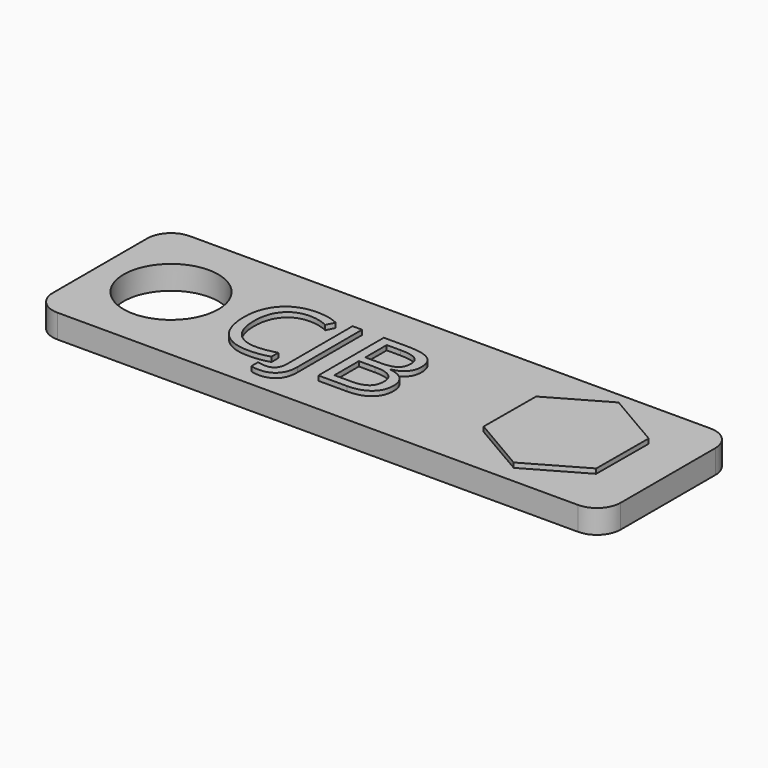
from build123d import *

# Parameters (mm, degrees)
F0_W         = 120
F0_H         = 35
F0_R         = 10
F1_DEPTH     = 5
F2_R         = 5
F3_TEXT_SIZE = 24.2037207095
F4_DEPTH     = 1


# Not quite as in the source:
# - Text() gives the source's letters only with a copy of the font that has no kerning and outlines rounded to 1/6400 em; it was checked with that copy


with BuildPart() as f1:
    # F0 (on Top) → F1 (new body)
    with BuildSketch(Plane.XY):
        Rectangle(F0_W, F0_H)
        with Locations((-45, 0)):
            Circle(F0_R, mode=Mode.SUBTRACT)
    extrude(amount=F1_DEPTH)

    # F2
    f2_edges = [f1.edges().sort_by_distance(p)[0] for p in [
        (60, -17.5, 2.5),
        (60, 17.5, 2.5),
        (-60, -17.5, 2.5),
        (-60, 17.5, 2.5),
    ]]
    fillet(f2_edges, radius=F2_R)

    # F3 (on face) → F4 (join)
    with BuildSketch(Plane.XY.offset(5)):
        Polygon((38.5482001709, 13.7803674473), (26.5833746983, 6.9433181749), (26.5220203188, -6.8370492723), (38.4254914118, -13.7803674473), (50.3903168844, -6.9433181749), (50.4516712639, 6.8370492723), align=None)
        with Locations((-30.2673876286, -9.6305338666)):
            Text('CJB', F3_TEXT_SIZE, font='Open Sans', text_align=(TextAlign.LEFT, TextAlign.BOTTOM))
    extrude(amount=F4_DEPTH)


solid = f1.part
